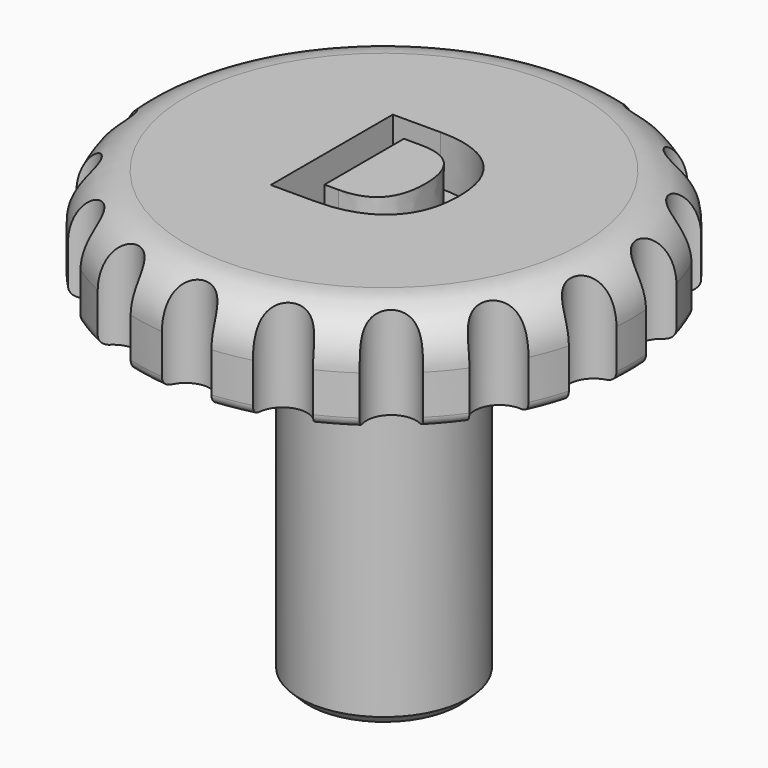
from build123d import *

# Parameters (mm, degrees)
F0_R         = 8.5
F0_W         = 10
F0_H         = 10
F1_DEPTH     = 35
F2_DEPTH     = 10
F3_SIZE      = 1
F4_R         = 25
F4_R_2       = 8.5
F5_DEPTH     = 10
F6_R         = 5
F8_R         = 1
F7_TEXT_SIZE = 21.5394939813
F9_DEPTH     = 5
F10_R        = 2.5
F11_DEPTH    = 25
F12_SIZE     = 0.9


# Not quite as in the source:
# - Text() gives the source's letters only with a copy of the font that has no kerning and outlines rounded to 1/6400 em; it was checked with that copy


with BuildPart() as f1:
    # F0 (on Top) → F1 (new body)
    with BuildSketch(Plane.XY):
        Circle(F0_R)
        Rectangle(F0_W, F0_H, mode=Mode.SUBTRACT)
        Rectangle(F0_W, F0_H)
    extrude(amount=F1_DEPTH)

    # F0 (on Top) → F2 (cut)
    with BuildSketch(Plane.XY):
        Rectangle(F0_W, F0_H)
    extrude(amount=F2_DEPTH, mode=Mode.SUBTRACT)

    # F3
    f3_edges = [f1.edges().sort_by_distance(p)[0] for p in [
        (-5, -5, 5),
        (-5, 5, 5),
        (5, 5, 5),
        (5, -5, 5),
    ]]
    chamfer(f3_edges, length=F3_SIZE)

    # F4 (on face) → F5 (join)
    with BuildSketch(Plane.XY.offset(35)):
        Circle(F4_R)
        Circle(F4_R_2, mode=Mode.SUBTRACT)
        Circle(F4_R)
    extrude(amount=F5_DEPTH)

    # F6
    f6_edges = [f1.edges().sort_by_distance(p)[0] for p in [
        (-8.5, 0, 35),
        (-25, 0, 45),
    ]]
    fillet(f6_edges, radius=F6_R)

    # F8
    f8_edges = [f1.edges().sort_by_distance(p)[0] for p in [
        (-25, 0, 35),
    ]]
    fillet(f8_edges, radius=F8_R)

    # F7 (on face) → F9 (cut)
    with BuildSketch(Plane.XY.offset(45)):
        with Locations((-7.3469867752, -7.503178902)):
            Text('D', F7_TEXT_SIZE, font='Open Sans', font_style=FontStyle.BOLD, text_align=(TextAlign.LEFT, TextAlign.BOTTOM))
    extrude(amount=-F9_DEPTH, mode=Mode.SUBTRACT)

    # F10 (on face) → F11 (cut)
    with BuildSketch(Plane.XY.offset(45)):
        with Locations((0, -25)):
            Circle(F10_R)
        with Locations((8.5505035831, -23.4923155196)):
            Circle(F10_R)
        with Locations((16.0696902422, -19.151111078)):
            Circle(F10_R)
        with Locations((21.6506350946, -12.5)):
            Circle(F10_R)
        with Locations((24.6201938253, -4.3412044417)):
            Circle(F10_R)
        with Locations((24.6201938253, 4.3412044417)):
            Circle(F10_R)
        with Locations((21.6506350946, 12.5)):
            Circle(F10_R)
        with Locations((16.0696902422, 19.151111078)):
            Circle(F10_R)
        with Locations((8.5505035831, 23.4923155196)):
            Circle(F10_R)
        with Locations((0, 25)):
            Circle(F10_R)
        with Locations((-8.5505035831, 23.4923155196)):
            Circle(F10_R)
        with Locations((-16.0696902422, 19.151111078)):
            Circle(F10_R)
        with Locations((-21.6506350946, 12.5)):
            Circle(F10_R)
        with Locations((-24.6201938253, 4.3412044417)):
            Circle(F10_R)
        with Locations((-24.6201938253, -4.3412044417)):
            Circle(F10_R)
        with Locations((-21.6506350946, -12.5)):
            Circle(F10_R)
        with Locations((-16.0696902422, -19.151111078)):
            Circle(F10_R)
        with Locations((-8.5505035831, -23.4923155196)):
            Circle(F10_R)
    extrude(amount=-F11_DEPTH, mode=Mode.SUBTRACT)

    # F12
    f12_edges = [f1.edges().sort_by_distance(p)[0] for p in [
        (-8.5, 0, 0),
    ]]
    chamfer(f12_edges, length=F12_SIZE)


solid = f1.part
